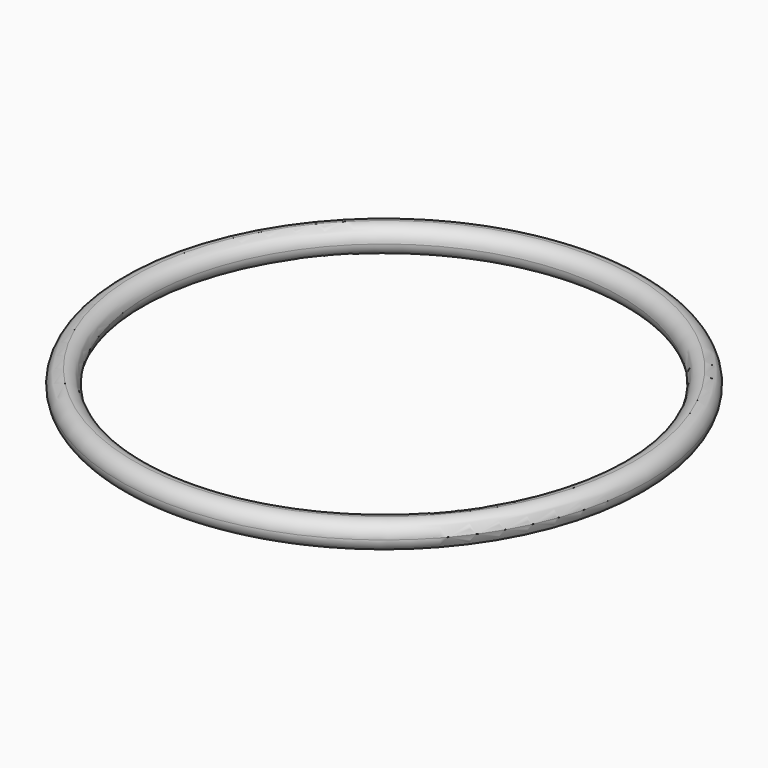
from build123d import *

# Parameters (mm, degrees)
F0_R     = 39
F0_R_2   = 35
F1_DEPTH = 4
F2_R     = 1.99999
F3_R     = 1.99999


# Not quite as in the source:
# - a fillet or chamfer is up to 0.001 mm smaller than in the source, because OpenCascade refuses the exact size


with BuildPart() as f1:
    # F0 (on Top) → F1 (new body)
    with BuildSketch(Plane.XY):
        Circle(F0_R)
        Circle(F0_R_2, mode=Mode.SUBTRACT)
    extrude(amount=F1_DEPTH)

    # F2 (radius 2 in the source; OpenCascade refuses exactly that, so slightly less here)
    f2_edges = [f1.edges().sort_by_distance(p)[0] for p in [
        (-39, 0, 0),
        (-35, 0, 0),
    ]]
    fillet(f2_edges, radius=F2_R)

    # F3 (radius 2 in the source; OpenCascade refuses exactly that, so slightly less here)
    f3_edges = [f1.edges().sort_by_distance(p)[0] for p in [
        (-39, 0, 4),
        (-35, 0, 4),
    ]]
    fillet(f3_edges, radius=F3_R)


solid = f1.part
